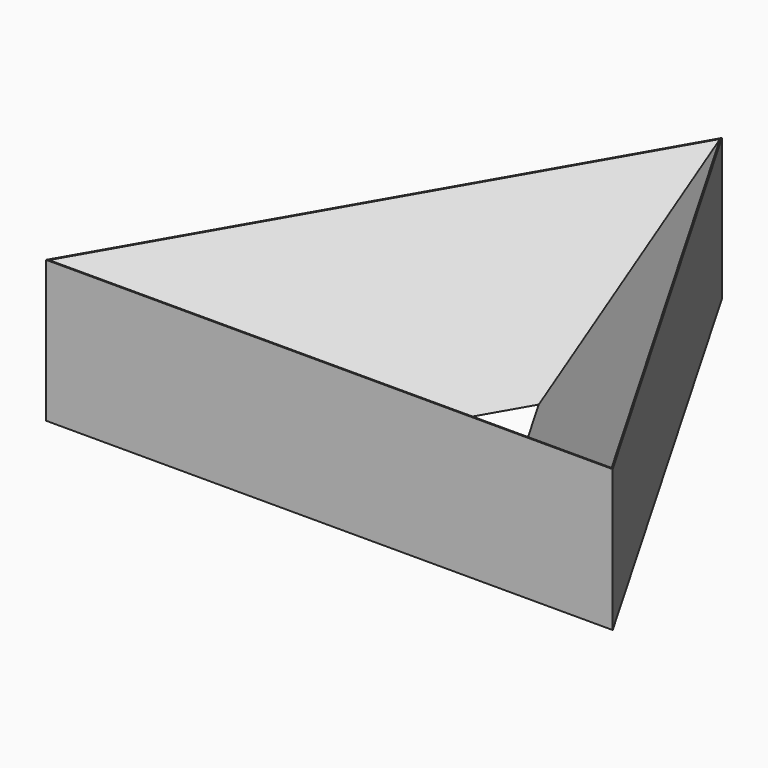
from build123d import *

# Parameters (mm, degrees)
F1_DEPTH = 12.7
F2_SIZE2 = 10.15999
F2_SIZE  = 12.69999


# Not quite as in the source:
# - a fillet or chamfer is up to 0.001 mm smaller than in the source, because OpenCascade refuses the exact size


with BuildPart() as f1:
    # F0 (on Top) → F1 (new body)
    with BuildSketch(Plane.XY):
        Polygon((0, 43.9940905122), (-25.4, 0), (-7.62, 10.2652877862), (0, 23.4635149399), align=None)
        Polygon((7.62, 10.2652877862), (25.4, 0), (0, 43.9940905122), (0, 23.4635149399), align=None)
        Polygon((-7.62, 10.2652877862), (-25.4, 0), (25.4, 0), (7.62, 10.2652877862), align=None)
    extrude(amount=F1_DEPTH)

    # F2 (size 12.7 and 10.16 in the source; OpenCascade refuses exactly that, so slightly less here)
    f2_edges = [f1.edges().sort_by_distance(p)[0] for p in [
        (0, 10.265288, 12.7),
        (-3.81, 16.864401, 12.7),
        (3.81, 16.864401, 12.7),
    ]]
    chamfer(f2_edges, length=F2_SIZE, length2=F2_SIZE2)


solid = f1.part
